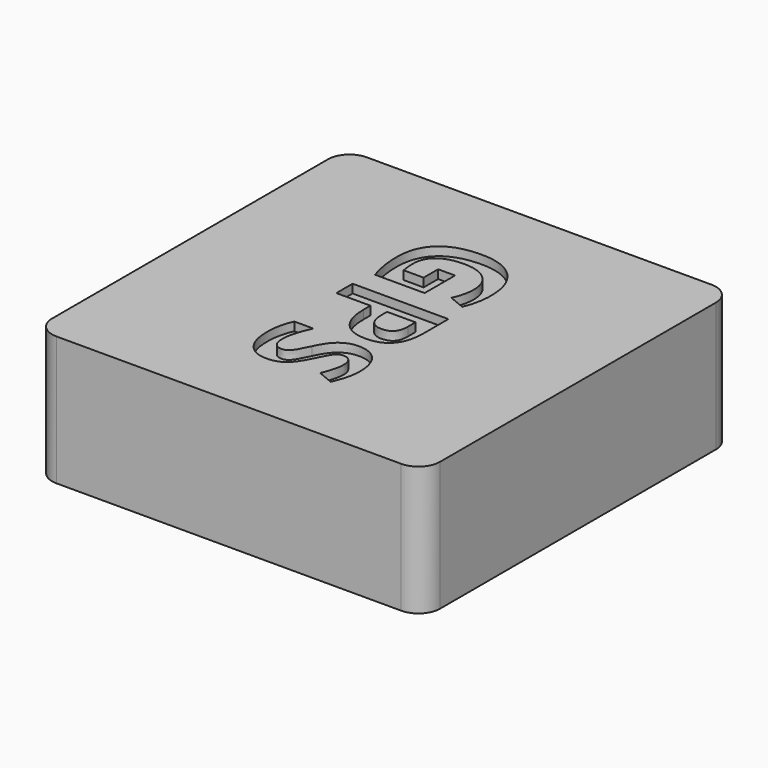
from build123d import *

# Parameters (mm, degrees)
F1_DEPTH     = 2
F2_TEXT_SIZE = 15.5591572123
F3_DEPTH     = 1
F4_W         = 39
F4_H         = 39
F5_DEPTH     = 13
F6_W         = 12
F6_H         = 6
F7_DEPTH     = 5


# Not quite as in the source:
# - Text() gives the source's letters only with a copy of the font that has no kerning and outlines rounded to 1/6400 em; it was checked with that copy


with BuildPart() as f1:
    # F0 (on Top) → F1 (new body)
    with BuildSketch(Plane.XY):
        with BuildLine():
            Line((20, 22.5), (-20, 22.5))
            ThreePointArc((-20, 22.5), (-21.767766953, 21.767766953), (-22.5, 20))
            Line((-22.5, 20), (-22.5, 10))
            Line((-22.5, 10), (-22.5, -10))
            Line((-22.5, -10), (-22.5, -20))
            ThreePointArc((-22.5, -20), (-21.767766953, -21.767766953), (-20, -22.5))
            Line((-20, -22.5), (20, -22.5))
            ThreePointArc((20, -22.5), (21.767766953, -21.767766953), (22.5, -20))
            Line((22.5, -20), (22.5, 20))
            ThreePointArc((22.5, 20), (21.767766953, 21.767766953), (20, 22.5))
        make_face()
    extrude(amount=F1_DEPTH)

    # F2 (on face) → F3 (cut)
    with BuildSketch(Plane.XY.offset(2)):
        with Locations(Location((-5.51, 15), (0, 0, -90))):
            Text('GPS', F2_TEXT_SIZE, font='Open Sans', font_style=FontStyle.BOLD, text_align=(TextAlign.LEFT, TextAlign.BOTTOM))
    extrude(amount=-F3_DEPTH, mode=Mode.SUBTRACT)

    # F4 (on face) → F5 (join)
    with BuildSketch(Plane(origin=(0, 0, 0), x_dir=(1, 0, 0), z_dir=(0, 0, -1))):
        with BuildLine():
            Line((20, 22.5), (-20, 22.5))
            ThreePointArc((-20, 22.5), (-21.767766953, 21.767766953), (-22.5, 20))
            Line((-22.5, 20), (-22.5, -20))
            ThreePointArc((-22.5, -20), (-21.767766953, -21.767766953), (-20, -22.5))
            Line((-20, -22.5), (20, -22.5))
            ThreePointArc((20, -22.5), (21.767766953, -21.767766953), (22.5, -20))
            Line((22.5, -20), (22.5, 20))
            ThreePointArc((22.5, 20), (21.767766953, 21.767766953), (20, 22.5))
        make_face()
        Rectangle(F4_W, F4_H, mode=Mode.SUBTRACT)
    extrude(amount=F5_DEPTH)

    # F6 (on face) → F7 (cut)
    with BuildSketch(Plane(origin=(-22.5, 0, 0), x_dir=(0, -1, 0), z_dir=(-1, 0, 0))):
        with Locations((-1.5, -10)):
            Rectangle(F6_W, F6_H)
    extrude(amount=-F7_DEPTH, mode=Mode.SUBTRACT)


solid = f1.part
